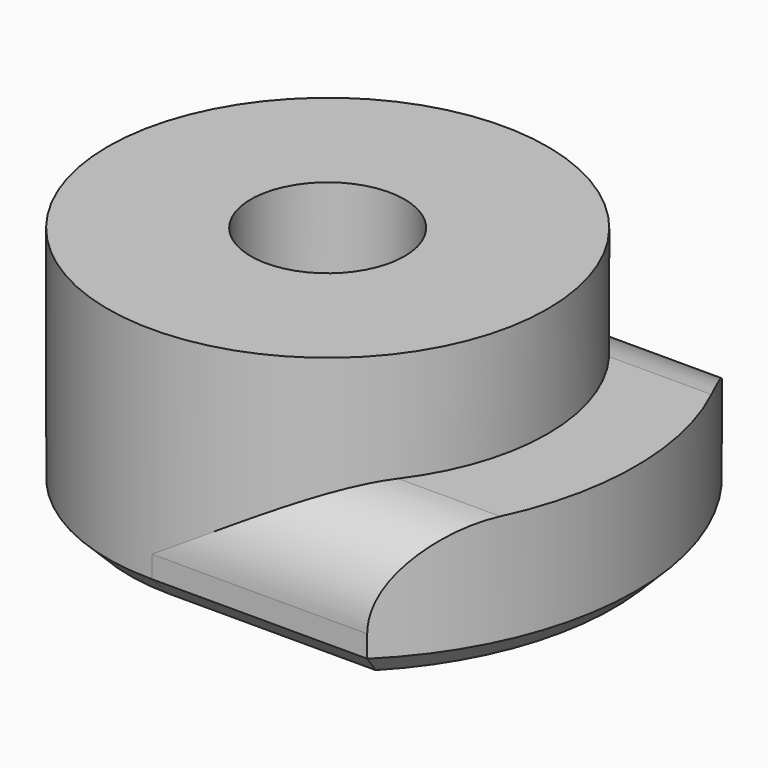
from build123d import *

# Parameters (mm, degrees)
F0_R         = 5
F0_R_2       = 1.75
F1_DEPTH     = 5.5
F3_DEPTH     = 3
F4_T4_DEPTH  = 14.8989794856
F4_S5_R      = 5
F4_T6_DEPTH  = 9
F4_T10_DEPTH = 14.8989794856
F4_S11_R     = 5
F4_T12_DEPTH = 9
F5_SIZE      = 0.5


# Not quite as in the source:
# - a fillet or chamfer that OpenCascade refuses, or shapes differently, is made with other operations: its cross-section is extruded or revolved along the edge and cut away or added


with BuildPart() as f1:
    # F0 (on Top) → F1 (new body)
    with BuildSketch(Plane.XY):
        Circle(F0_R)
        Circle(F0_R_2, mode=Mode.SUBTRACT)
    extrude(amount=F1_DEPTH)

    # F2 (on Top) → F3 (join)
    with BuildSketch(Plane.XY):
        with BuildLine():
            Line((0, -5), (4.8989794856, -5))
            ThreePointArc((4.8989794856, -5), (7, 0), (4.8989794856, 5))
            Line((4.8989794856, 5), (0, 5))
            ThreePointArc((0, 5), (5, 0), (0, -5))
        make_face()
    extrude(amount=F3_DEPTH)

    # F4: fillet of radius 2 on 2 edges, made by hand


with BuildPart() as f4_tool2:
    # F4_s3 → F4_t4 (new body)
    with BuildSketch(Plane.YZ.offset(-5)):
        with BuildLine():
            ThreePointArc((-3, 3), (-4.4142135624, 2.4142135624), (-5, 1))
            Line((-5, 1), (-5, 3))
            Line((-5, 3), (-3, 3))
        make_face()
    extrude(amount=F4_T4_DEPTH)

    # F4_s5 → F4_t6 (cut, symmetric)
    with BuildSketch(Plane.XY.offset(2)):
        Circle(F4_S5_R)
    extrude(amount=F4_T6_DEPTH, both=True, mode=Mode.SUBTRACT)


with BuildPart() as f1_1:
    add(f1.part)

    # F4_t1: cut F4_tool2
    add(f4_tool2.part, mode=Mode.SUBTRACT)


with BuildPart() as f4_tool8:
    # F4_s9 → F4_t10 (new body)
    with BuildSketch(Plane.YZ.offset(9.8989794856)):
        with BuildLine():
            ThreePointArc((3, 3), (4.4142135624, 2.4142135624), (5, 1))
            Line((5, 1), (5, 3))
            Line((5, 3), (3, 3))
        make_face()
    extrude(amount=-F4_T10_DEPTH)

    # F4_s11 → F4_t12 (cut, symmetric)
    with BuildSketch(Plane.XY.offset(2)):
        Circle(F4_S11_R)
    extrude(amount=F4_T12_DEPTH, both=True, mode=Mode.SUBTRACT)


with BuildPart() as f1_2:
    add(f1_1.part)

    # F4_t7: cut F4_tool8
    add(f4_tool8.part, mode=Mode.SUBTRACT)

    # F5
    f5_edges = [f1_2.edges().sort_by_distance(p)[0] for p in [
        (-5, 0, 0),
        (2.44949, -5, 0),
        (7, 0, 0),
        (2.44949, 5, 0),
        (-1.75, 0, 0),
    ]]
    chamfer(f5_edges, length=F5_SIZE)


solid = f1_2.part
